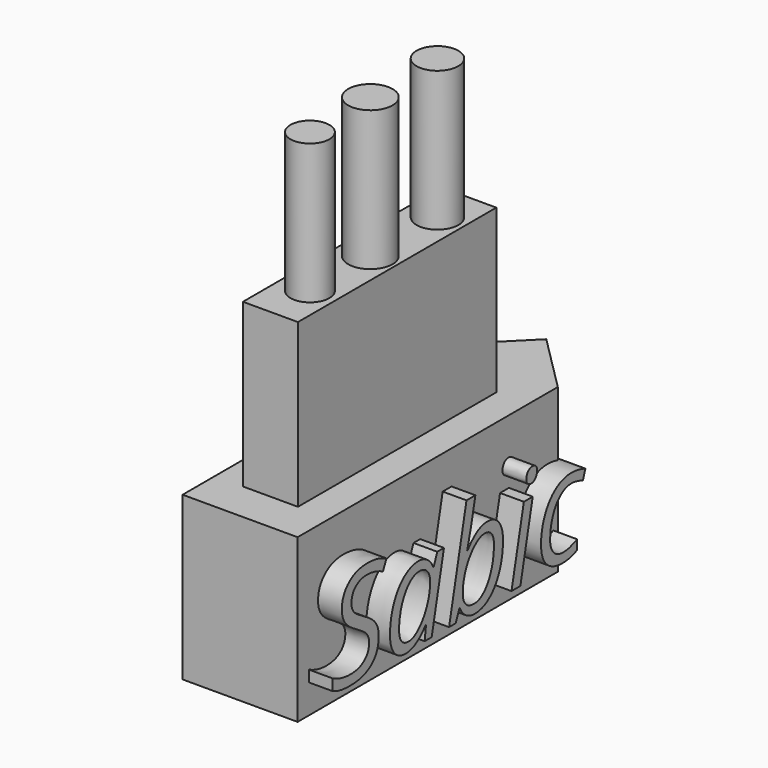
from build123d import *

# Parameters (mm, degrees)
F1_DEPTH     = 25.4
F2_W         = 8.5915257223
F2_H         = 38.7223716825
F3_DEPTH     = 25.4
F4_R         = 3.2648463684
F4_R_2       = 3.0415581386
F4_R_3       = 3.4663934779
F5_DEPTH     = 72.644
F6_TEXT_SIZE = 21.1192605396
F7_DEPTH     = 12.7


# Not quite as in the source:
# - Text() gives the source's letters only with a copy of the font that has no kerning and outlines rounded to 1/6400 em; it was checked with that copy


with BuildPart() as f1:
    # F0 (on Top) → F1 (new body)
    with BuildSketch(Plane.XY):
        Polygon((-8.9802561211, 22.5587171747), (-8.9802561211, -28.2412828253), (8.9802561211, -28.2412828253), (8.9802561211, 22.5587171747), (0, 31.5389732958), align=None)
    extrude(amount=F1_DEPTH)

    # F2 (on face) → F3 (join)
    with BuildSketch(Plane.XY.offset(25.4)):
        with Locations((-0.2943777945, -2.5894725695)):
            Rectangle(F2_W, F2_H)
    extrude(amount=F3_DEPTH)

    # F4 (on Top) → F5 (join)
    with BuildSketch(Plane.XY):
        with Locations((0, 10.286022909)):
            Circle(F4_R)
        with Locations((0, -14.6091766655)):
            Circle(F4_R_2)
        with Locations((0, -2.8091396671)):
            Circle(F4_R_3)
    extrude(amount=F5_DEPTH)

    # F6 (on Right) → F7 (join)
    with BuildSketch(Plane.YZ):
        with Locations((-26.4634899795, 4.1108243167)):
            Text('Sabic', F6_TEXT_SIZE, font='Open Sans', font_style=FontStyle.ITALIC, text_align=(TextAlign.LEFT, TextAlign.BOTTOM))
    extrude(amount=F7_DEPTH)


solid = f1.part
